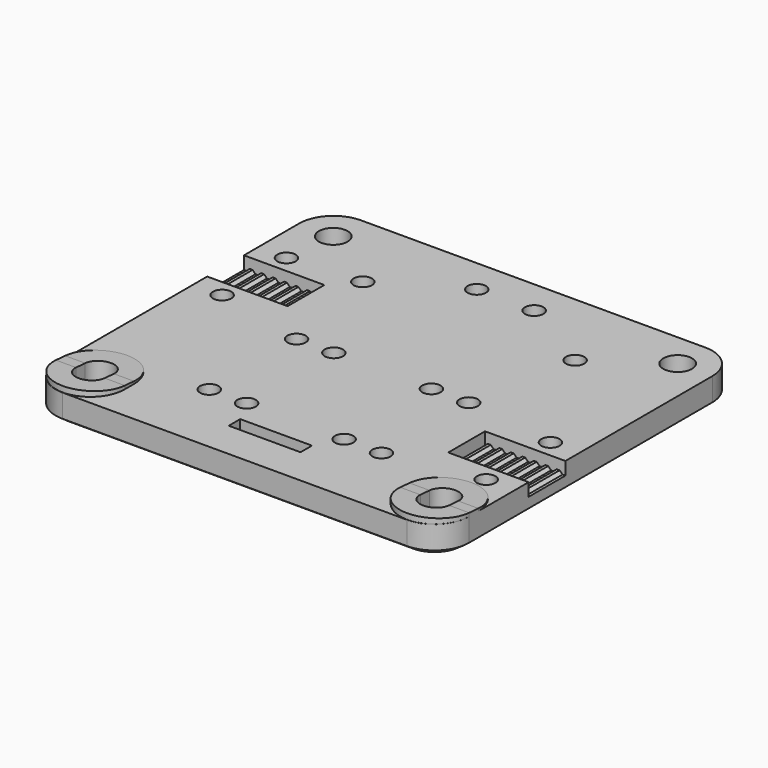
from build123d import *

# Parameters (mm, degrees)
F0_W      = 72
F0_H      = 65
F0_R      = 2.5
F1_DEPTH  = 5
F2_R      = 6
F3_W      = 14
F3_H      = 8
F4_DEPTH  = 2.25
F3_R      = 1.6
F5_DEPTH  = 2
F7_DEPTH  = 2.9
F8_DEPTH  = 1
F10_DEPTH = 72.001
F12_DEPTH = 8
F14_DEPTH = 8
F3_W_2    = 12.5
F3_H_2    = 2.5
F15_DEPTH = 5.001
F16_SIZE2 = 3
F16_SIZE  = 3
F17_SIZE2 = 0.9802905535
F17_SIZE  = 1.4


# Not quite as in the source:
# - ends of sketch curves that miss each other by under 0.0002 mm in the source are joined


with BuildPart() as f1:
    # F0 (on Top) → F1 (new body)
    with BuildSketch(Plane.XY):
        Rectangle(F0_W, F0_H)
        with BuildLine():
            Line((-32.4999988079, -26.449996978), (-32.4999988079, -24.4499966502))
            ThreePointArc((-32.4999988079, -24.4499966502), (-30, -21.9499978423), (-27.5000011921, -24.4499966502))
            Line((-27.5000011921, -24.4499966502), (-27.5000011921, -26.449996978))
            ThreePointArc((-27.5000011921, -26.449996978), (-30, -28.949995786), (-32.4999988079, -26.449996978))
        make_face(mode=Mode.SUBTRACT)
        with BuildLine():
            Line((27.5000044703, -26.4499968141), (27.5000044703, -24.4499968141))
            ThreePointArc((27.5000044703, -24.4499968141), (30, -21.9499968141), (32.5, -24.4499968141))
            Line((32.5, -24.4499968141), (32.5, -26.4499968141))
            ThreePointArc((32.5, -26.4499968141), (30, -28.9499968141), (27.5000044703, -26.4499968141))
        make_face(mode=Mode.SUBTRACT)
        with Locations((-30, 26.45)):
            Circle(F0_R, mode=Mode.SUBTRACT)
        with Locations((30, 26.45)):
            Circle(F0_R, mode=Mode.SUBTRACT)
    extrude(amount=F1_DEPTH)

    # F2
    f2_edges = [f1.edges().sort_by_distance(p)[0] for p in [
        (-36, 32.5, 2.5),
        (36, 32.5, 2.5),
        (36, -32.5, 2.5),
        (-36, -32.5, 2.5),
    ]]
    fillet(f2_edges, radius=F2_R)

    # F3 (on face) → F4 (cut)
    with BuildSketch(Plane.XY.offset(5)):
        with Locations((-29, 10.5)):
            Rectangle(F3_W, F3_H)
        with Locations((29, -9.4999990389)):
            Rectangle(F3_W, F3_H)
    extrude(amount=-F4_DEPTH, mode=Mode.SUBTRACT)

    # F3 (on face) → F5 (cut)
    with BuildSketch(Plane.XY.offset(5)):
        with Locations((5, 26.45)):
            Circle(F3_R)
        with Locations((-5, 26.45)):
            Circle(F3_R)
        with Locations((-31, 17.5)):
            Circle(F3_R)
        with Locations((-31, 3.5)):
            Circle(F3_R)
        with Locations((31, -2.4999990389)):
            Circle(F3_R)
        with Locations((31, -16.4999990389)):
            Circle(F3_R)
        with Locations((-15, -0.3)):
            Circle(F3_R)
        with Locations((-8.5, -0.3)):
            Circle(F3_R)
        with Locations((8.5, -0.3)):
            Circle(F3_R)
        with Locations((15, -0.3)):
            Circle(F3_R)
        with Locations((15, -19.3)):
            Circle(F3_R)
        with Locations((8.5, -19.3)):
            Circle(F3_R)
        with Locations((-8.5, -19.3)):
            Circle(F3_R)
        with Locations((-15, -19.3)):
            Circle(F3_R)
        with Locations((-18.5, 18.5)):
            Circle(F3_R)
        with Locations((18.5, 18.5)):
            Circle(F3_R)
    extrude(amount=-F5_DEPTH, mode=Mode.SUBTRACT)

    # F6 (on face) → F7 (cut)
    with BuildSketch(Plane.XY):
        Polygon((-29.3256842193, 20.4), (-32.6743157807, 20.4), (-34.3486315613, 17.5), (-32.6743157806, 14.6), (-29.3256842193, 14.6), (-27.6513684387, 17.5), align=None)
        Polygon((-29.3256842194, 6.4), (-32.6743157807, 6.4), (-34.3486315613, 3.5), (-32.6743157806, 0.6), (-29.3256842194, 0.6), (-27.6513684387, 3.5), align=None)
        Polygon((-6.6743157806, 23.55), (-3.3256842194, 23.55), (-1.6513684387, 26.45), (-3.3256842194, 29.35), (-6.6743157806, 29.35), (-8.3486315613, 26.45), align=None)
        Polygon((3.3256842194, 23.55), (6.6743157806, 23.55), (8.3486315613, 26.45), (6.6743157806, 29.35), (3.3256842194, 29.35), (1.6513684387, 26.45), align=None)
        Polygon((29.3256842194, -5.3999990389), (32.6743157807, -5.3999990389), (34.3486315613, -2.4999990389), (32.6743157806, 0.4000009611), (29.3256842194, 0.4000009611), (27.6513684387, -2.4999990389), align=None)
        Polygon((34.3486315613, -16.4999990389), (32.6743157807, -13.5999990389), (29.3256842194, -13.5999990389), (27.6513684387, -16.4999990389), (29.3256842193, -19.3999990389), (32.6743157806, -19.3999990389), align=None)
        Polygon((-12.1, -20.9743157806), (-12.1, -17.6256842194), (-15, -15.9513684387), (-17.9, -17.6256842194), (-17.9, -20.9743157806), (-15, -22.6486315613), align=None)
        Polygon((-11.4, -17.6256842193), (-11.4, -20.9743157807), (-8.5, -22.6486315613), (-5.6, -20.9743157806), (-5.6, -17.6256842193), (-8.5, -15.9513684387), align=None)
        Polygon((11.4, -20.6965663945), (11.4, -17.9034336055), (9.2162408508, -16.1619437962), (6.4931377323, -16.7834743131), (5.2812428339, -19.3), (6.4931377323, -21.8165256869), (9.2162408508, -22.4380562038), align=None)
        Polygon((18.2187571661, -19.3), (17.0068622677, -16.7834743131), (14.2837591492, -16.1619437962), (12.1, -17.9034336055), (12.1, -20.6965663945), (14.2837591492, -22.4380562038), (17.0068622677, -21.8165256869), align=None)
        Polygon((12.1, 1.3743157806), (12.1, -1.9743157806), (15, -3.6486315613), (17.9, -1.9743157806), (17.9, 1.3743157806), (15, 3.0486315613), align=None)
        Polygon((11.4, -1.9743157807), (11.4, 1.3743157807), (8.5, 3.0486315613), (5.6, 1.3743157806), (5.6, -1.9743157807), (8.5, -3.6486315613), align=None)
        Polygon((-11.4, 1.3743157807), (-11.4, -1.9743157807), (-8.5, -3.6486315613), (-5.6, -1.9743157806), (-5.6, 1.3743157807), (-8.5, 3.0486315613), align=None)
        Polygon((-12.1, -1.9743157807), (-12.1, 1.3743157807), (-15, 3.0486315613), (-17.9, 1.3743157806), (-17.9, -1.9743157807), (-15, -3.6486315613), align=None)
        Polygon((16.8256842194, 15.6), (20.1743157806, 15.6), (21.8486315613, 18.5), (20.1743157806, 21.4), (16.8256842194, 21.4), (15.1513684387, 18.5), align=None)
        Polygon((-20.1743157806, 15.6), (-16.8256842194, 15.6), (-15.1513684387, 18.5), (-16.8256842194, 21.4), (-20.1743157806, 21.4), (-21.8486315613, 18.5), align=None)
    extrude(amount=F7_DEPTH, mode=Mode.SUBTRACT)

    # F3 (on face) → F8 (join)
    with BuildSketch(Plane.XY.offset(5)):
        with BuildLine():
            Line((36, -26.4499968141), (36, -24.4499968141))
            ThreePointArc((36, -24.4499968141), (30, -18.4499968141), (24, -24.4499968141))
            Line((24, -24.4499968141), (24.0000044703, -26.4499968141))
            ThreePointArc((24.0000044703, -26.4499968141), (30, -32.4499968141), (36, -26.4499968141))
        make_face()
        with BuildLine():
            ThreePointArc((32.5, -26.4499968141), (30.0000022351, -28.9499968141), (27.5000044703, -26.4499968141))
            Line((27.5000044703, -26.4499968141), (27.5000044703, -24.4499968141))
            ThreePointArc((27.5000044703, -24.4499968141), (30.0000022351, -21.9499968141), (32.5, -24.4499968141))
            Line((32.5, -24.4499968141), (32.5, -26.4499968141))
        make_face(mode=Mode.SUBTRACT)
        with BuildLine():
            ThreePointArc((-24.0000011921, -24.4499966502), (-30, -18.4499978423), (-35.9999988079, -24.4499966502))
            Line((-35.9999988079, -24.4499966502), (-36, -26.449996978))
            ThreePointArc((-36, -26.449996978), (-30, -32.449995786), (-24.0000011921, -26.449996978))
            Line((-24.0000011921, -26.449996978), (-24.0000011921, -24.4499966502))
        make_face()
        with BuildLine():
            ThreePointArc((-27.5000011921, -26.449996978), (-30, -28.949995786), (-32.4999988079, -26.449996978))
            Line((-32.4999988079, -26.449996978), (-32.4999988079, -24.4499966502))
            ThreePointArc((-32.4999988079, -24.4499966502), (-30, -21.9499978423), (-27.5000011921, -24.4499966502))
            Line((-27.5000011921, -24.4499966502), (-27.5000011921, -26.449996978))
        make_face(mode=Mode.SUBTRACT)
    extrude(amount=F8_DEPTH)

    # F9 (on face) → F10 (cut, through all)
    with BuildSketch(Plane.YZ.offset(36)):
        Polygon((-26.4499968141, 5.5714285714), (-24.4499968141, 5.4285714286), (-24.4499968141, 6), (-26.4499968141, 6), align=None)
        Polygon((-24.4499968141, 5.4285714286), (-18.4499968141, 5), (-18.4499968141, 6), (-24.4499968141, 6), align=None)
        Polygon((-32.4499968141, 6), (-26.4499968141, 5.5714285714), (-26.4499968141, 6), align=None)
    extrude(amount=-F10_DEPTH, mode=Mode.SUBTRACT)

    # F11 (on face) → F12 (join, through all)
    with BuildSketch(Plane.XZ.offset(-14.5)):
        Polygon((-35, 3.25), (-35.5, 2.75), (-34, 2.75), (-34.5, 3.25), align=None)
        Polygon((-33, 3.25), (-33.5, 2.75), (-32, 2.75), (-32.5, 3.25), align=None)
        Polygon((-31, 3.25), (-31.5, 2.75), (-30, 2.75), (-30.5, 3.25), align=None)
        Polygon((-29, 3.25), (-29.5, 2.75), (-28, 2.75), (-28.5, 3.25), align=None)
        Polygon((-27.5, 2.75), (-26, 2.75), (-26.5, 3.25), (-27, 3.25), align=None)
        Polygon((-25.5, 2.75), (-24, 2.75), (-24.5, 3.25), (-25, 3.25), align=None)
        Polygon((-23.5, 2.75), (-22, 2.75), (-22.5, 3.25), (-23, 3.25), align=None)
    extrude(amount=F12_DEPTH)

    # F13 (on face) → F14 (join, through all)
    with BuildSketch(Plane(origin=(0, -13.4999990389, 0), x_dir=(-1, 0, 0), z_dir=(0, 1, 0))):
        Polygon((-25.5, 2.75), (-24, 2.75), (-24.5, 3.25), (-25, 3.25), align=None)
        Polygon((-27.5, 2.75), (-26, 2.75), (-26.5, 3.25), (-27, 3.25), align=None)
        Polygon((-23.5, 2.75), (-22, 2.75), (-22.5, 3.25), (-23, 3.25), align=None)
        Polygon((-29, 3.25), (-29.5, 2.75), (-28, 2.75), (-28.5, 3.25), align=None)
        Polygon((-31, 3.25), (-31.5, 2.75), (-30, 2.75), (-30.5, 3.25), align=None)
        Polygon((-33, 3.25), (-33.5, 2.75), (-32, 2.75), (-32.5, 3.25), align=None)
        Polygon((-35, 3.25), (-35.5, 2.75), (-34, 2.75), (-34.5, 3.25), align=None)
    extrude(amount=F14_DEPTH)

    # F3 (on face) → F15 (cut, through all)
    with BuildSketch(Plane.XY.offset(5)):
        with Locations((0, -24.75)):
            Rectangle(F3_W_2, F3_H_2)
    extrude(amount=-F15_DEPTH, mode=Mode.SUBTRACT)

    # F16
    f16_edges = [f1.edges().sort_by_distance(p)[0] for p in [
        (0, -26, 0),
    ]]
    chamfer(f16_edges, length=F16_SIZE, length2=F16_SIZE2)

    # F17
    f17_edges = [f1.edges().sort_by_distance(p)[0] for p in [
        (0, -32.5, 0),
    ]]
    f17_side = f1.faces().sort_by_distance((0.004579, 0.46074, 0))[0]
    chamfer(f17_edges, length=F17_SIZE, length2=F17_SIZE2, reference=f17_side)


solid = f1.part
